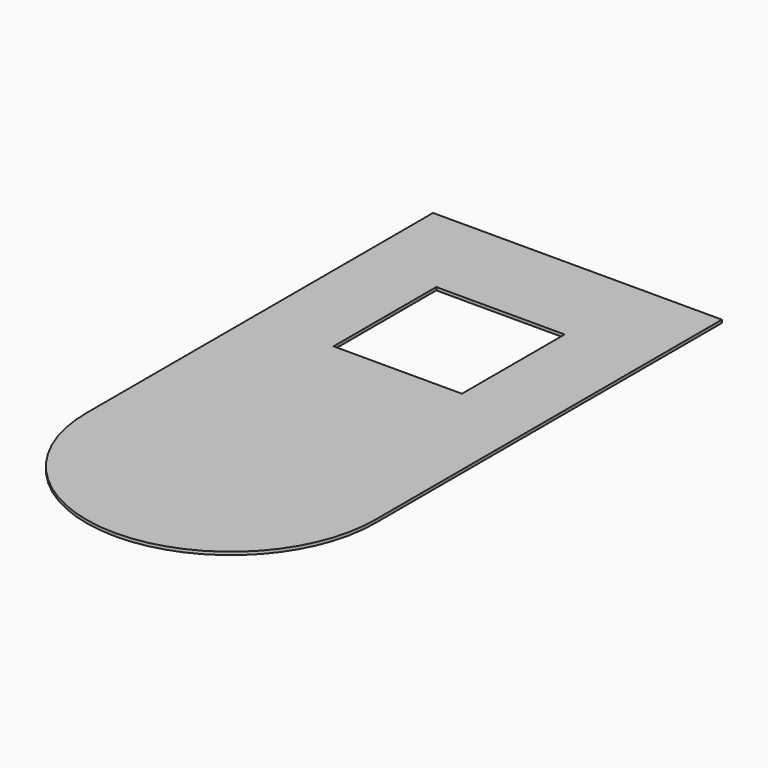
from build123d import *

# Parameters (mm, degrees)
F0_W     = 457.2
F0_H     = 914.4
F1_DEPTH = 4.7752
F2_R     = 228.59999
F3_W     = 203.2
F3_H     = 203.2
F4_DEPTH = 25.399999693


# Not quite as in the source:
# - a fillet or chamfer is up to 0.001 mm smaller than in the source, because OpenCascade refuses the exact size
# - ends of sketch curves that miss each other by under 0.0002 mm in the source are joined


with BuildPart() as f1:
    # F0 (on Top) → F1 (new body)
    with BuildSketch(Plane.XY):
        with Locations((0, 457.2)):
            Rectangle(F0_W, F0_H)
    extrude(amount=F1_DEPTH)

    # F2 (radius 228.6 in the source; OpenCascade refuses exactly that, so slightly less here)
    f2_edges = [f1.edges().sort_by_distance(p)[0] for p in [
        (228.6, 0, 2.3876),
        (-228.6, 0, 2.3876),
    ]]
    fillet(f2_edges, radius=F2_R)

    # F3 (on face) → F4 (intersect)
    with BuildSketch(Plane.XY.offset(4.7752)):
        with BuildLine():
            Line((-228.6, 914.4), (-228.6, 228.59999))
            ThreePointArc((-228.6, 228.59999), (-161.6446131082, 66.9553868918), (-1e-05, 0))
            ThreePointArc((-1e-05, 0), (161.6446131082, 66.9553868918), (228.6, 228.59999))
            Line((228.6, 228.59999), (228.6, 914.4))
            Line((228.6, 914.4), (-228.6, 914.4))
        make_face()
        with Locations((0, 660.4)):
            Rectangle(F3_W, F3_H, mode=Mode.SUBTRACT)
    extrude(amount=-F4_DEPTH, mode=Mode.INTERSECT)


solid = f1.part
